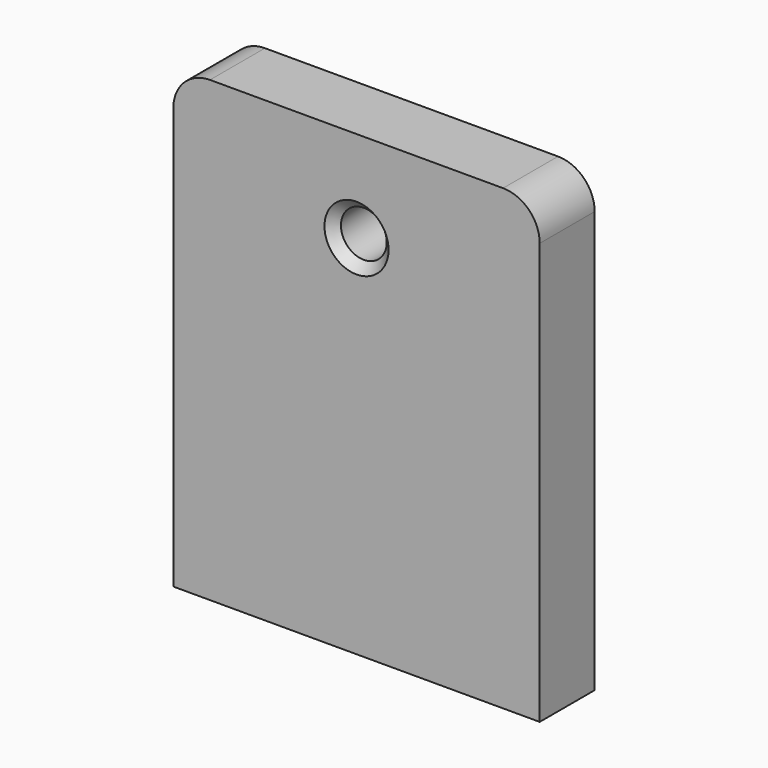
from build123d import *

# Parameters (mm, degrees)
F0_W     = 50.8
F0_H     = 9.525
F1_DEPTH = 63.5
F2_R     = 3.175
F3_DEPTH = 9.525
F4_R     = 3.175
F5_DEPTH = 12.7
F6_R     = 5.08
F7_SIZE  = 1.27


# Not quite as in the source:
# - a length typed as a fraction of an inch, garbled in the dataset ("3 / 203.2 mm" for 3/8 in), is restored


with BuildPart() as f1:
    # F0 (on Top) → F1 (new body)
    with BuildSketch(Plane.XY):
        with Locations((-25.4, 4.7625)):
            Rectangle(F0_W, F0_H)
    extrude(amount=F1_DEPTH)

    # F2 (on face) → F3 (cut)
    with BuildSketch(Plane.XZ):
        with Locations((-25.4, 50.8)):
            Circle(F2_R)
    extrude(amount=-F3_DEPTH, mode=Mode.SUBTRACT)

    # F4 (on face) → F5 (cut)
    with BuildSketch(Plane(origin=(0, 0, 0), x_dir=(1, 0, 0), z_dir=(0, 0, -1))):
        with Locations((-38.1, -4.7625)):
            Circle(F4_R)
        with Locations((-12.7, -4.7625)):
            Circle(F4_R)
    extrude(amount=-F5_DEPTH, mode=Mode.SUBTRACT)

    # F6
    f6_edges = [f1.edges().sort_by_distance(p)[0] for p in [
        (-50.8, 4.7625, 63.5),
        (0, 4.7625, 63.5),
    ]]
    fillet(f6_edges, radius=F6_R)

    # F7
    f7_edges = [f1.edges().sort_by_distance(p)[0] for p in [
        (-28.575, 0, 50.8),
        (-28.575, 9.525, 50.8),
    ]]
    chamfer(f7_edges, length=F7_SIZE)


solid = f1.part
